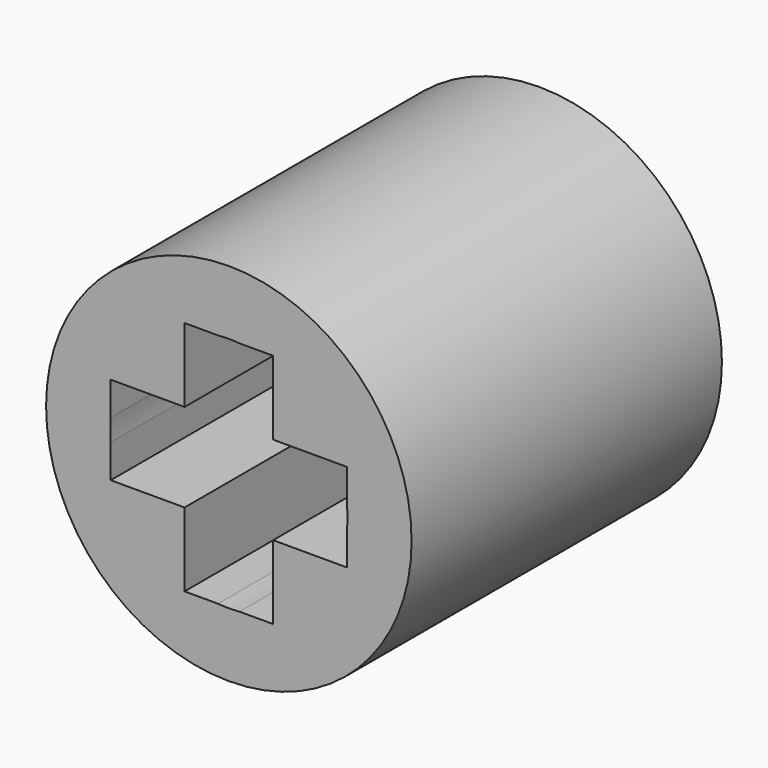
from build123d import *

# Parameters (mm, degrees)
F0_R     = 3.675
F1_DEPTH = 7.8
F2_DEPTH = 7.8


# Not quite as in the source:
# - a feature names something its author has since deleted; it is built from what else it names


with BuildPart() as f1:
    # F0 (on Front) → F1 (new body)
    with BuildSketch(Plane.XZ):
        Circle(F0_R)
        with BuildLine():
            Line((-2.375, 0.2181742423), (-2.375, 0.89))
            Line((-2.375, 0.89), (-2.2127189157, 0.89))
            ThreePointArc((-2.2127189157, 0.89), (-1.6864496731, 1.6864496731), (-0.89, 2.2127189157))
            Line((-0.89, 2.2127189157), (-0.89, 2.375))
            Line((-0.89, 2.375), (-0.2181742423, 2.375))
            ThreePointArc((-0.2181742423, 2.375), (0, 2.385), (0.2181742423, 2.375))
            Line((0.2181742423, 2.375), (0.89, 2.375))
            Line((0.89, 2.375), (0.89, 2.2127189157))
            ThreePointArc((0.89, 2.2127189157), (1.6864496731, 1.6864496731), (2.2127189157, 0.89))
            Line((2.2127189157, 0.89), (2.375, 0.89))
            Line((2.375, 0.89), (2.375, 0.2181742423))
            ThreePointArc((2.375, 0.2181742423), (2.3824986884, 0.1092016483), (2.385, 0))
            ThreePointArc((2.385, 0), (2.3824986884, -0.1092016483), (2.375, -0.2181742423))
            Line((2.375, -0.2181742423), (2.375, -0.89))
            Line((2.375, -0.89), (2.2127189157, -0.89))
            ThreePointArc((2.2127189157, -0.89), (1.6864496731, -1.6864496731), (0.89, -2.2127189157))
            Line((0.89, -2.2127189157), (0.89, -2.375))
            Line((0.89, -2.375), (0.2181742423, -2.375))
            ThreePointArc((0.2181742423, -2.375), (0, -2.385), (-0.2181742423, -2.375))
            Line((-0.2181742423, -2.375), (-0.89, -2.375))
            Line((-0.89, -2.375), (-0.89, -2.2127189157))
            ThreePointArc((-0.89, -2.2127189157), (-1.6864496731, -1.6864496731), (-2.2127189157, -0.89))
            Line((-2.2127189157, -0.89), (-2.375, -0.89))
            Line((-2.375, -0.89), (-2.375, -0.2181742423))
            ThreePointArc((-2.375, -0.2181742423), (-2.385, 0), (-2.375, 0.2181742423))
        make_face(mode=Mode.SUBTRACT)
    extrude(amount=F1_DEPTH)

    # F0 (on Front) → F2 (join)
    with BuildSketch(Plane.XZ):
        with BuildLine():
            ThreePointArc((-0.89, 2.2127189157), (-1.6864496731, 1.6864496731), (-2.2127189157, 0.89))
            Line((-2.2127189157, 0.89), (-0.89, 0.89))
            Line((-0.89, 0.89), (-0.89, 2.2127189157))
        make_face()
        with BuildLine():
            Line((0.89, 2.2127189157), (0.89, 0.89))
            Line((0.89, 0.89), (2.2127189157, 0.89))
            ThreePointArc((2.2127189157, 0.89), (1.6864496731, 1.6864496731), (0.89, 2.2127189157))
        make_face()
        with BuildLine():
            Line((-0.89, -0.89), (-2.2127189157, -0.89))
            ThreePointArc((-2.2127189157, -0.89), (-1.6864496731, -1.6864496731), (-0.89, -2.2127189157))
            Line((-0.89, -2.2127189157), (-0.89, -0.89))
        make_face()
        with BuildLine():
            Line((2.2127189157, -0.89), (0.89, -0.89))
            Line((0.89, -0.89), (0.89, -2.2127189157))
            ThreePointArc((0.89, -2.2127189157), (1.6864496731, -1.6864496731), (2.2127189157, -0.89))
        make_face()
    extrude(amount=F2_DEPTH)


solid = f1.part
